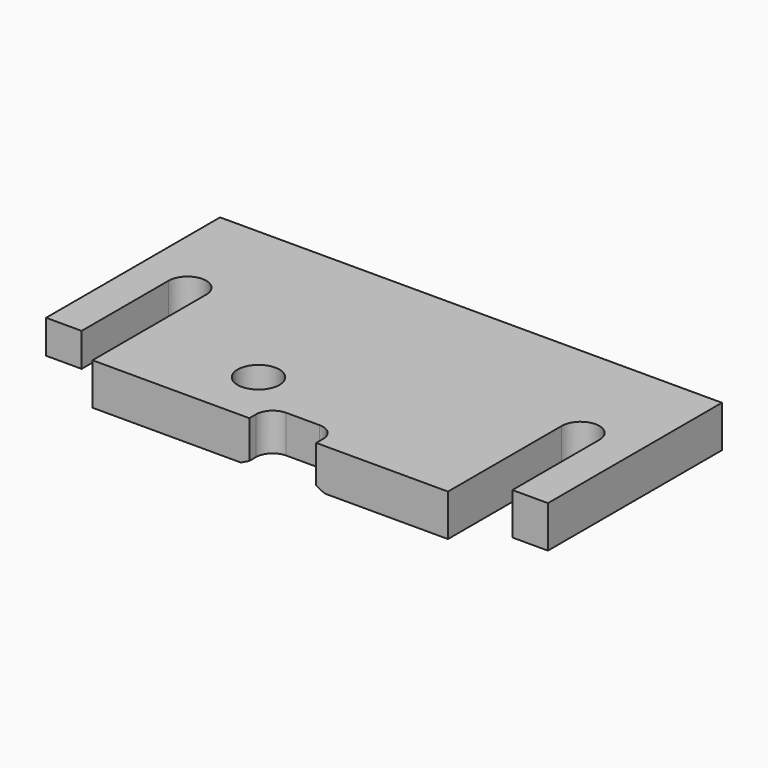
from build123d import *

# Parameters (mm, degrees)
F1_DEPTH = 5
F2_D     = 5
F3_SIZE2 = 0.5
F3_SIZE  = 1
F4_W     = 4.25
F4_H     = 26
F5_DEPTH = 1


with BuildPart() as f1:
    # F0 (on Top) → F1 (new body)
    with BuildSketch(Plane.XY):
        with BuildLine():
            Line((60, 0), (0, 0))
            Line((0, 0), (0, -26))
            Line((0, -26), (4.25, -26))
            Line((4.25, -26), (4.25, -13))
            ThreePointArc((4.25, -13), (6.5, -10.75), (8.75, -13))
            Line((8.75, -13), (8.75, -30))
            Line((8.75, -30), (27.5, -30))
            Line((27.5, -30), (27.5, -29))
            ThreePointArc((27.5, -29), (28.0857864376, -27.5857864376), (29.5, -27))
            Line((29.5, -27), (33.5, -27))
            ThreePointArc((33.5, -27), (34.9142135624, -27.5857864376), (35.5, -29))
            Line((35.5, -29), (35.5, -30))
            Line((35.5, -30), (51.25, -30))
            Line((51.25, -30), (51.25, -13))
            ThreePointArc((51.25, -13), (53.5, -10.75), (55.75, -13))
            Line((55.75, -13), (55.75, -26))
            Line((55.75, -26), (60, -26))
            Line((60, -26), (60, 0))
        make_face()
    extrude(amount=-F1_DEPTH)

    # F2 (through all)
    with Locations(Plane.XY):
        with Locations((23, -23)):
            Hole(F2_D / 2)

    # F3
    f3_edges = [f1.edges().sort_by_distance(p)[0] for p in [
        (31.5, -27, -5),
    ]]
    f3_side = f1.faces().sort_by_distance((30.066886, -13.81093, -5))[0]
    chamfer(f3_edges, length=F3_SIZE, length2=F3_SIZE2, reference=f3_side)

    # F4 (on face) → F5 (cut)
    with BuildSketch(Plane(origin=(0, 0, -5), x_dir=(1, 0, 0), z_dir=(0, 0, -1))):
        with Locations((2.125, 13)):
            Rectangle(F4_W, F4_H)
    extrude(amount=-F5_DEPTH, mode=Mode.SUBTRACT)


solid = f1.part
